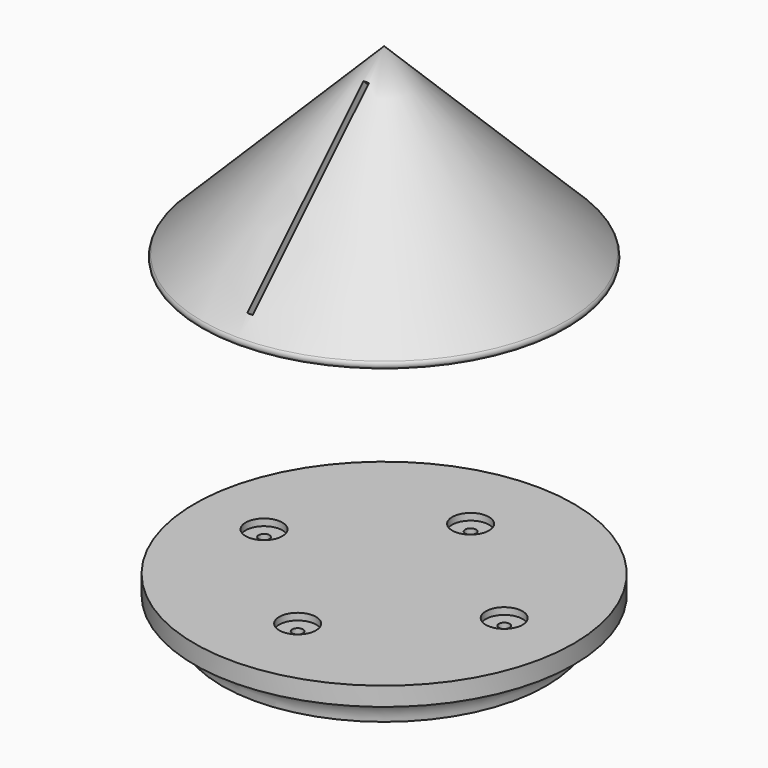
from build123d import *

# Parameters (mm, degrees)
F3_D           = 5
F3_CBORE_D     = 17
F3_CBORE_DEPTH = 3.15
F5_D           = 5
F5_CBORE_D     = 17
F5_CBORE_DEPTH = 3.1496
F7_D           = 4
F7_DEPTH       = 3.1496
F7_CBORE_D     = 17
F7_CBORE_DEPTH = 3.1496
F7_TIP         = 1.2017212381
F12_ANGLE      = 25
F14_R          = 8.5
F15_DEPTH      = 12.39
F16_R          = 2
F18_W          = 2.5
F18_H          = 95
F19_DEPTH      = 10


with BuildPart() as f1:
    # F0 (on Front) → F1 (revolve)
    with BuildSketch(Plane.XZ):
        with BuildLine():
            Line((0, 21.3487), (0, 0))
            Line((0, 0), (74.93, 0))
            ThreePointArc((74.93, 0), (78.6497438789, 8.9802561211), (87.63, 12.7))
            Line((87.63, 12.7), (87.63, 21.3487))
            Line((87.63, 21.3487), (0, 21.3487))
        make_face()
    revolve(axis=Axis((0, 0, 10.67435), (0, 0, -1)))

    # F3 (through all)
    with Locations(Plane.XY.offset(21.3487)):
        with Locations((-55.5371, 0), (55.5371, 0)):
            CounterBoreHole(F3_D / 2, F3_CBORE_D / 2, F3_CBORE_DEPTH)

    # F5 (through all)
    with Locations(Plane.XY.offset(21.3487)):
        with Locations((0, 50), (0, -50)):
            CounterBoreHole(F5_D / 2, F5_CBORE_D / 2, F5_CBORE_DEPTH)

    # F7
    with Locations(Plane(origin=(0, 0, 0), x_dir=(1, 0, 0), z_dir=(0, 0, -1))):
        with Locations((0, 50), (0, -50)):
            CounterBoreHole(F7_D / 2, F7_CBORE_D / 2, F7_CBORE_DEPTH, depth=F7_DEPTH)
            with Locations((0, 0, -(F7_DEPTH + F7_TIP / 2))):  # 118° drill point
                Cone(0, F7_D / 2, F7_TIP, mode=Mode.SUBTRACT)


with BuildPart() as f11:
    # F10 (on Right) → F11 (revolve)
    with BuildSketch(Plane.YZ):
        Polygon((-52.5, 157.2387), (-52.5, 148.3487), (-47.5, 148.3487), (-47.5, 157.2387), (-45, 157.2387), (-45, 160.7387), (-50, 160.7387), (-55, 160.7387), (-55, 157.2387), align=None)
        Polygon((-87.8178626299, 148.3487), (-52.5, 148.3487), (-52.5, 157.2387), (-55, 157.2387), (-55, 160.7387), (-50, 160.7387), (-45, 160.7387), (-45, 157.2387), (-47.5, 157.2387), (-47.5, 148.3487), (0, 148.3487), (0, 236.1665626299), align=None)
    revolve(axis=Axis((0, 0, 192.2576313149), (0, 0, 1)))


with BuildPart() as f12:
    # F10 (on Right) → F12 (revolve)
    with BuildSketch(Plane.YZ):
        Polygon((-52.5, 157.2387), (-52.5, 148.3487), (-47.5, 148.3487), (-47.5, 157.2387), (-45, 157.2387), (-45, 160.7387), (-50, 160.7387), (-55, 160.7387), (-55, 157.2387), align=None)
    revolve(axis=Axis((0, 0, 192.2576313149), (0, 0, -1)), revolution_arc=F12_ANGLE)


with BuildPart() as f12b:
    # F10 (on Right) → F12, piece 2 (revolve)
    with BuildSketch(Plane.YZ):
        Polygon((55, 160.7387), (50, 160.7387), (45, 160.7387), (45, 157.2387), (47.5, 157.2387), (47.5, 148.3487), (52.5, 148.3487), (52.5, 157.2387), (55, 157.2387), align=None)
    revolve(axis=Axis((0, 0, 192.2576313149), (0, 0, -1)), revolution_arc=F12_ANGLE)


with BuildPart() as f11_1:
    add(f11.part)

    # F13: cut F12, F12b
    add(f12.part, mode=Mode.SUBTRACT)
    add(f12b.part, mode=Mode.SUBTRACT)

    # F14 (on face) → F15 (cut, through all)
    with BuildSketch(Plane(origin=(0, 0, 148.3487), x_dir=(1, 0, 0), z_dir=(0, 0, -1))):
        with Locations((0, -50)):
            Circle(F14_R)
        with Locations((0, 50)):
            Circle(F14_R)
    extrude(amount=-F15_DEPTH, mode=Mode.SUBTRACT)

    # F16
    f16_edges = [f11_1.edges().sort_by_distance(p)[0] for p in [
        (0, 87.817863, 148.3487),
    ]]
    fillet(f16_edges, radius=F16_R)

    # F18 (on face) → F19 (cut)
    with BuildSketch(Plane(origin=(0, -118.0832813149, 118.0832813149), x_dir=(1, 0, 0), z_dir=(0, -0.7071067812, 0.7071067812))):
        with Locations((0, 104.8017655753)):
            Rectangle(F18_W, F18_H)
    extrude(amount=-F19_DEPTH, mode=Mode.SUBTRACT)


solid = Compound([f1.part, f11_1.part])
